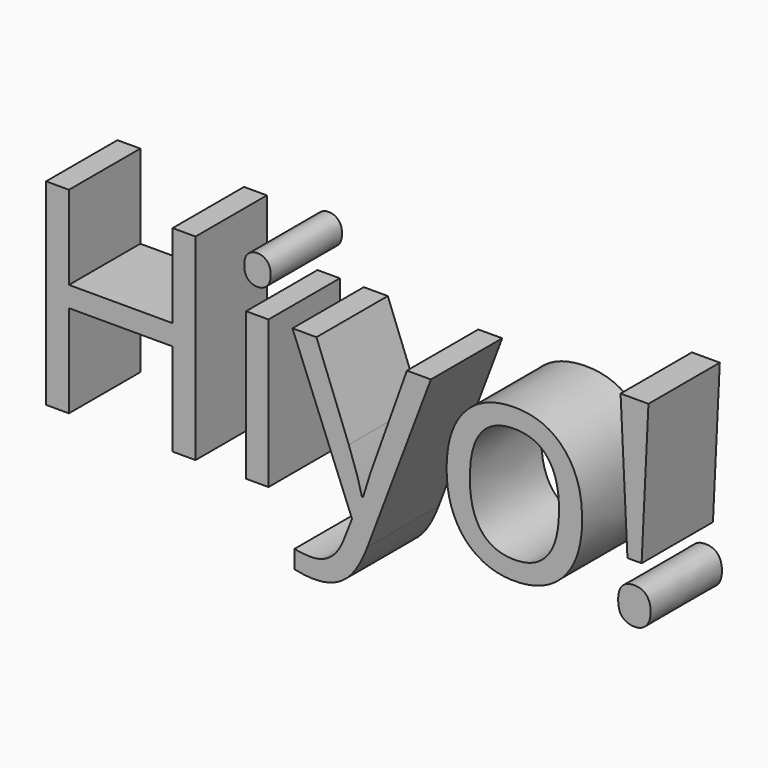
from build123d import *

# Parameters (mm, degrees)
F0_TEXT_SIZE = 157.0649652017
F1_DEPTH     = 50.8


# Not quite as in the source:
# - Text() gives the source's letters only with a copy of the font that has no kerning and outlines rounded to 1/6400 em; it was checked with that copy


with BuildPart() as f1:
    # F0 (on Front) → F1 (new body)
    with BuildSketch(Plane.XZ):
        with Locations((-201.0431662202, -64.2538480461)):
            Text('Hiyo!', F0_TEXT_SIZE, font='Open Sans', text_align=(TextAlign.LEFT, TextAlign.BOTTOM))
    extrude(amount=F1_DEPTH)


solid = f1.part
